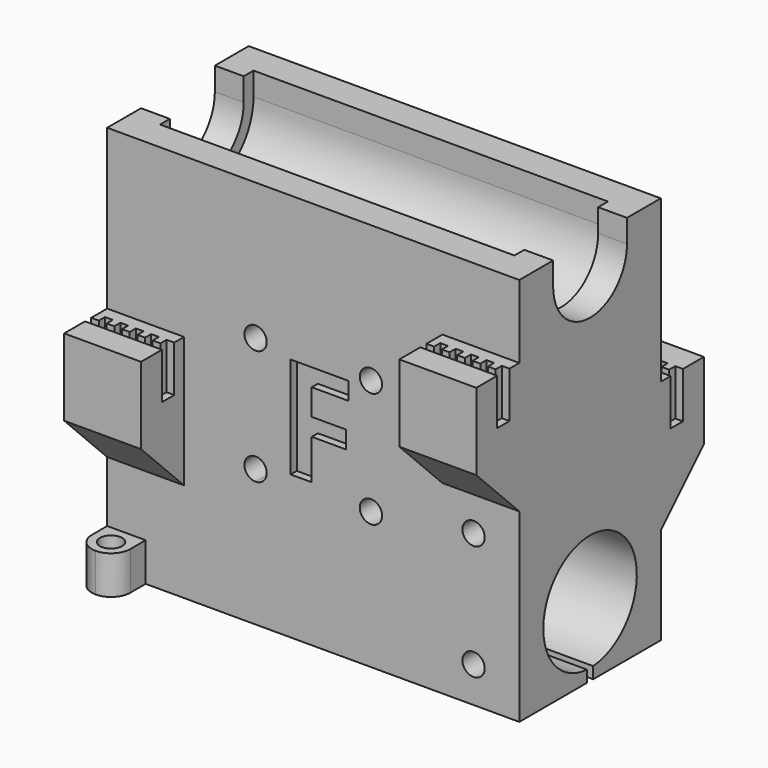
from build123d import *

# Parameters (mm, degrees)
F1_W          = 53.6
F1_H          = 23
F2_DEPTH      = 50.6
F4_DEPTH      = 53.601
F5_DEPTH      = 49.85
F6_DEPTH      = 24.95
F7_DEPTH      = 25.05
F8_DEPTH      = 3.75
F9_W          = 10
F9_H          = 20
F10_DEPTH     = 7
F11_T4_DEPTH  = 61.4336597593
F11_T9_DEPTH  = 61.4336597593
F13_DEPTH     = 6
F15_DEPTH     = 6
F16_W         = 10
F16_H         = 20
F17_DEPTH     = 7
F19_DEPTH     = 6
F21_DEPTH     = 6
F22_T4_DEPTH  = 61.4336597593
F22_T9_DEPTH  = 61.4336597593
F23_R         = 1.45
F24_DEPTH     = 30.001
F25_R         = 1.45
F26_DEPTH     = 5
F27_TEXT_SIZE = 18.4411155982
F28_DEPTH     = 1
F29_W         = 5
F29_H         = 5
F30_DEPTH     = 5
F31_R         = 1.45
F32_DEPTH     = 25
F33_R         = 2.49999


# Not quite as in the source:
# - a fillet or chamfer that OpenCascade refuses, or shapes differently, is made with other operations: its cross-section is extruded or revolved along the edge and cut away or added
# - a fillet or chamfer is up to 0.001 mm smaller than in the source, because OpenCascade refuses the exact size
# - a feature names something its author has since deleted; it is built from what else it names
# - Text() gives the source's letters only with a copy of the font that has no kerning and outlines rounded to 1/6400 em; it was checked with that copy


with BuildPart() as f2:
    # F1 (on Top) → F2 (new body)
    with BuildSketch(Plane.XY):
        with Locations((26.8, 11.5)):
            Rectangle(F1_W, F1_H)
    extrude(amount=F2_DEPTH)

    # F3 (on face) → F4 (cut, through all)
    with BuildSketch(Plane(origin=(0, 0, 0), x_dir=(0, -1, 0), z_dir=(-1, 0, 0))):
        with BuildLine():
            ThreePointArc((-11, 1.5164652041), (-11.5, 1.5), (-12, 1.5164652041))
            Line((-12, 1.5164652041), (-12, 0))
            Line((-12, 0), (-11.5, 0))
            Line((-11.5, 0), (-11, 0))
            Line((-11, 0), (-11, 1.5164652041))
        make_face()
        with BuildLine():
            Line((-11, 1.5164652041), (-12, 1.5164652041))
            ThreePointArc((-12, 1.5164652041), (-11.5, 1.5), (-11, 1.5164652041))
        make_face()
        with BuildLine():
            ThreePointArc((-11, 1.5164652041), (-5.9520273973, 3.9057724347), (-3.9, 9.1))
            ThreePointArc((-3.9, 9.1), (-16.6942275653, 14.6479726027), (-12, 1.5164652041))
            Line((-12, 1.5164652041), (-11, 1.5164652041))
        make_face()
        with BuildLine():
            Line((-5.5, 47.6), (-5.5, 50.6))
            Line((-5.5, 50.6), (-6.3038475773, 50.6))
            ThreePointArc((-6.3038475773, 50.6), (-5.7044450423, 49.1529142706), (-5.5, 47.6))
        make_face()
        with BuildLine():
            Line((-16.6961524227, 50.6), (-17.5, 50.6))
            Line((-17.5, 50.6), (-17.5, 47.6))
            ThreePointArc((-17.5, 47.6), (-17.2955549577, 49.1529142706), (-16.6961524227, 50.6))
        make_face()
        with BuildLine():
            ThreePointArc((-16.6961524227, 50.6), (-17.2955549577, 49.1529142706), (-17.5, 47.6))
            ThreePointArc((-17.5, 47.6), (-11.5, 41.6), (-5.5, 47.6))
            ThreePointArc((-5.5, 47.6), (-5.7044450423, 49.1529142706), (-6.3038475773, 50.6))
            Line((-6.3038475773, 50.6), (-16.6961524227, 50.6))
        make_face()
    extrude(amount=-F4_DEPTH, mode=Mode.SUBTRACT)

    # F3 (on face) → F5 (cut)
    with BuildSketch(Plane(origin=(0, 0, 0), x_dir=(0, -1, 0), z_dir=(-1, 0, 0))):
        with BuildLine():
            ThreePointArc((-18.4828361, 50.6), (-18.9441102343, 49.1314120346), (-19.1, 47.6))
            ThreePointArc((-19.1, 47.6), (-11.5, 40), (-3.9, 47.6))
            ThreePointArc((-3.9, 47.6), (-4.0558897657, 49.1314120346), (-4.5171639, 50.6))
            Line((-4.5171639, 50.6), (-5.5, 50.6))
            Line((-5.5, 50.6), (-5.5, 47.6))
            ThreePointArc((-5.5, 47.6), (-11.5, 41.6), (-17.5, 47.6))
            Line((-17.5, 47.6), (-17.5, 50.6))
            Line((-17.5, 50.6), (-18.4828361, 50.6))
        make_face()
        with BuildLine():
            Line((-18.4828361, 50.6), (-19.1, 50.6))
            Line((-19.1, 50.6), (-19.1, 47.6))
            ThreePointArc((-19.1, 47.6), (-18.9441102343, 49.1314120346), (-18.4828361, 50.6))
        make_face()
        with BuildLine():
            Line((-3.9, 47.6), (-3.9, 50.6))
            Line((-3.9, 50.6), (-4.5171639, 50.6))
            ThreePointArc((-4.5171639, 50.6), (-4.0558897657, 49.1314120346), (-3.9, 47.6))
        make_face()
    extrude(amount=-F5_DEPTH, mode=Mode.SUBTRACT)

    # F3 (on face) → F6 (join)
    with BuildSketch(Plane(origin=(0, 0, 0), x_dir=(0, -1, 0), z_dir=(-1, 0, 0))):
        with BuildLine():
            ThreePointArc((-18.4828361, 50.6), (-18.9441102343, 49.1314120346), (-19.1, 47.6))
            ThreePointArc((-19.1, 47.6), (-11.5, 40), (-3.9, 47.6))
            ThreePointArc((-3.9, 47.6), (-4.0558897657, 49.1314120346), (-4.5171639, 50.6))
            Line((-4.5171639, 50.6), (-5.5, 50.6))
            Line((-5.5, 50.6), (-5.5, 47.6))
            ThreePointArc((-5.5, 47.6), (-11.5, 41.6), (-17.5, 47.6))
            Line((-17.5, 47.6), (-17.5, 50.6))
            Line((-17.5, 50.6), (-18.4828361, 50.6))
        make_face()
        with BuildLine():
            Line((-18.4828361, 50.6), (-19.1, 50.6))
            Line((-19.1, 50.6), (-19.1, 47.6))
            ThreePointArc((-19.1, 47.6), (-18.9441102343, 49.1314120346), (-18.4828361, 50.6))
        make_face()
        with BuildLine():
            Line((-3.9, 47.6), (-3.9, 50.6))
            Line((-3.9, 50.6), (-4.5171639, 50.6))
            ThreePointArc((-4.5171639, 50.6), (-4.0558897657, 49.1314120346), (-3.9, 47.6))
        make_face()
    extrude(amount=-F6_DEPTH)

    # F3 (on face) → F7 (cut)
    with BuildSketch(Plane(origin=(0, 0, 0), x_dir=(0, -1, 0), z_dir=(-1, 0, 0))):
        with BuildLine():
            ThreePointArc((-18.4828361, 50.6), (-18.9441102343, 49.1314120346), (-19.1, 47.6))
            ThreePointArc((-19.1, 47.6), (-11.5, 40), (-3.9, 47.6))
            ThreePointArc((-3.9, 47.6), (-4.0558897657, 49.1314120346), (-4.5171639, 50.6))
            Line((-4.5171639, 50.6), (-5.5, 50.6))
            Line((-5.5, 50.6), (-5.5, 47.6))
            ThreePointArc((-5.5, 47.6), (-11.5, 41.6), (-17.5, 47.6))
            Line((-17.5, 47.6), (-17.5, 50.6))
            Line((-17.5, 50.6), (-18.4828361, 50.6))
        make_face()
        with BuildLine():
            Line((-18.4828361, 50.6), (-19.1, 50.6))
            Line((-19.1, 50.6), (-19.1, 47.6))
            ThreePointArc((-19.1, 47.6), (-18.9441102343, 49.1314120346), (-18.4828361, 50.6))
        make_face()
        with BuildLine():
            Line((-3.9, 47.6), (-3.9, 50.6))
            Line((-3.9, 50.6), (-4.5171639, 50.6))
            ThreePointArc((-4.5171639, 50.6), (-4.0558897657, 49.1314120346), (-3.9, 47.6))
        make_face()
    extrude(amount=-F7_DEPTH, mode=Mode.SUBTRACT)

    # F3 (on face) → F8 (join)
    with BuildSketch(Plane(origin=(0, 0, 0), x_dir=(0, -1, 0), z_dir=(-1, 0, 0))):
        with BuildLine():
            ThreePointArc((-18.4828361, 50.6), (-18.9441102343, 49.1314120346), (-19.1, 47.6))
            ThreePointArc((-19.1, 47.6), (-11.5, 40), (-3.9, 47.6))
            ThreePointArc((-3.9, 47.6), (-4.0558897657, 49.1314120346), (-4.5171639, 50.6))
            Line((-4.5171639, 50.6), (-5.5, 50.6))
            Line((-5.5, 50.6), (-5.5, 47.6))
            ThreePointArc((-5.5, 47.6), (-11.5, 41.6), (-17.5, 47.6))
            Line((-17.5, 47.6), (-17.5, 50.6))
            Line((-17.5, 50.6), (-18.4828361, 50.6))
        make_face()
        with BuildLine():
            Line((-18.4828361, 50.6), (-19.1, 50.6))
            Line((-19.1, 50.6), (-19.1, 47.6))
            ThreePointArc((-19.1, 47.6), (-18.9441102343, 49.1314120346), (-18.4828361, 50.6))
        make_face()
        with BuildLine():
            Line((-3.9, 47.6), (-3.9, 50.6))
            Line((-3.9, 50.6), (-4.5171639, 50.6))
            ThreePointArc((-4.5171639, 50.6), (-4.0558897657, 49.1314120346), (-3.9, 47.6))
        make_face()
    extrude(amount=-F8_DEPTH)

    # F9 (on face) → F10 (join)
    with BuildSketch(Plane.XZ):
        with Locations((5, 19.9)):
            Rectangle(F9_W, F9_H)
        with Locations((48.6, 31.1)):
            Rectangle(F9_W, F9_H)
    extrude(amount=F10_DEPTH)

    # F11: chamfer of 10 on 2 edges, made by hand


with BuildPart() as f11_tool2:
    # F11_s3 → F11_t4 (new body)
    with BuildSketch(Plane.YZ.offset(-25.7168298797)):
        Polygon((3, 9.9), (-7, 19.9), (-7, 9.9), align=None)
    extrude(amount=F11_T4_DEPTH)

    split(bisect_by=Plane.XZ, keep=Keep.TOP)


with BuildPart() as f2_1:
    add(f2.part)

    # F11_t1: cut F11_tool2
    add(f11_tool2.part, mode=Mode.SUBTRACT)


with BuildPart() as f11_tool7:
    # F11_s8 → F11_t9 (new body)
    with BuildSketch(Plane.YZ.offset(17.8831701203)):
        Polygon((3, 21.1), (-7, 31.1), (-7, 21.1), align=None)
    extrude(amount=F11_T9_DEPTH)

    split(bisect_by=Plane.XZ, keep=Keep.TOP)


with BuildPart() as f2_2:
    add(f2_1.part)

    # F11_t6: cut F11_tool7
    add(f11_tool7.part, mode=Mode.SUBTRACT)

    # F12 (on face) → F13 (cut)
    with BuildSketch(Plane.XY.offset(29.9)):
        Polygon((0, -2.6), (0, -3.6), (10, -3.6), (10, -2.6), (10, -1.6), (9, -1.6), (9, -2.6), (8, -2.6), (8, -1.6), (7, -1.6), (7, -2.6), (6, -2.6), (6, -1.6), (5.2958247252, -1.6), (5, -1.6), (5, -2.6), (4, -2.6), (4, -1.6), (3, -1.6), (3, -2.6), (2, -2.6), (2, -1.6), (1, -1.6), (1, -2.6), align=None)
    extrude(amount=-F13_DEPTH, mode=Mode.SUBTRACT)

    # F14 (on face) → F15 (cut)
    with BuildSketch(Plane.XY.offset(41.1)):
        Polygon((43.6, -2.6), (43.6, -3.6), (53.6, -3.6), (53.6, -2.6), (53.6, -1.6), (52.6, -1.6), (52.6, -2.6), (51.6, -2.6), (51.6, -1.6), (50.6, -1.6), (50.6, -2.6), (49.6, -2.6), (49.6, -1.6), (48.8349036932, -1.6), (48.6, -1.6), (48.6, -2.6), (47.6, -2.6), (47.6, -1.6), (46.6, -1.6), (46.6, -2.6), (45.6, -2.6), (45.6, -1.6), (44.6, -1.6), (44.6, -2.6), align=None)
    extrude(amount=-F15_DEPTH, mode=Mode.SUBTRACT)

    # F16 (on face) → F17 (join)
    with BuildSketch(Plane(origin=(0, 23, 0), x_dir=(-1, 0, 0), z_dir=(0, 1, 0))):
        with Locations((-48.6, 19.6)):
            Rectangle(F16_W, F16_H)
        with Locations((-5, 31.1)):
            Rectangle(F16_W, F16_H)
    extrude(amount=F17_DEPTH)

    # F18 (on face) → F19 (cut)
    with BuildSketch(Plane.XY.offset(29.6)):
        Polygon((43.6, 25.6), (43.6, 24.6), (48.6, 24.6), (53.6, 24.6), (53.6, 25.6), (53.6, 26.6), (52.6, 26.6), (52.6, 25.6), (51.6, 25.6), (51.6, 26.6), (50.6, 26.6), (50.6, 25.6), (49.6, 25.6), (49.6, 26.6), (48.6, 26.6), (48.6, 25.6), (47.6, 25.6), (47.6, 26.6), (46.6, 26.6), (46.6, 25.6), (45.6, 25.6), (45.6, 26.6), (44.6, 26.6), (44.6, 25.6), align=None)
    extrude(amount=-F19_DEPTH, mode=Mode.SUBTRACT)

    # F20 (on face) → F21 (cut)
    with BuildSketch(Plane.XY.offset(41.1)):
        Polygon((7, 25.6), (6, 25.6), (6, 26.6), (5, 26.6), (5, 25.6), (4, 25.6), (4, 26.6), (3, 26.6), (3, 25.6), (2, 25.6), (2, 26.6), (1, 26.6), (1, 25.6), (0, 25.6), (0, 24.6), (5, 24.6), (10, 24.6), (10, 25.6), (10, 26.6), (9, 26.6), (9, 25.6), (8, 25.6), (8, 26.6), (7, 26.6), align=None)
    extrude(amount=-F21_DEPTH, mode=Mode.SUBTRACT)

    # F22: chamfer of 10 on 2 edges, made by hand


with BuildPart() as f22_tool2:
    # F22_s3 → F22_t4 (new body)
    with BuildSketch(Plane.YZ.offset(35.7168298797)):
        Polygon((30, 31.1), (20, 21.1), (30, 21.1), align=None)
    extrude(amount=-F22_T4_DEPTH)

    split(bisect_by=Plane.XZ.offset(-23), keep=Keep.BOTTOM)


with BuildPart() as f2_3:
    add(f2_2.part)

    # F22_t1: cut F22_tool2
    add(f22_tool2.part, mode=Mode.SUBTRACT)


with BuildPart() as f22_tool7:
    # F22_s8 → F22_t9 (new body)
    with BuildSketch(Plane.YZ.offset(79.3168298797)):
        Polygon((20, 9.6), (30, 19.6), (30, 9.6), align=None)
    extrude(amount=-F22_T9_DEPTH)

    split(bisect_by=Plane.XZ.offset(-23), keep=Keep.BOTTOM)


with BuildPart() as f2_4:
    add(f2_3.part)

    # F22_t6: cut F22_tool7
    add(f22_tool7.part, mode=Mode.SUBTRACT)

    # F23 (on face) → F24 (cut, through all)
    with BuildSketch(Plane.XZ):
        with BuildLine():
            ThreePointArc((17.85, 32.8), (19.3, 31.35), (20.75, 32.8))
            ThreePointArc((20.75, 32.8), (19.3, 34.25), (17.85, 32.8))
        make_face()
        with BuildLine():
            ThreePointArc((35.75, 32.8), (35.3253048327, 33.8253048327), (34.3, 34.25))
            ThreePointArc((34.3, 34.25), (33.2746951673, 31.7746951673), (35.75, 32.8))
        make_face()
        with BuildLine():
            ThreePointArc((20.75, 17.8), (18.2746951673, 18.8253048327), (19.3, 16.35))
            ThreePointArc((19.3, 16.35), (20.3253048327, 16.7746951673), (20.75, 17.8))
        make_face()
        with Locations((34.3, 17.8)):
            Circle(F23_R)
    extrude(amount=-F24_DEPTH, mode=Mode.SUBTRACT)

    # F25 (on face) → F26 (cut)
    with BuildSketch(Plane.XZ):
        with Locations((47.65, 19.65)):
            Circle(F25_R)
        with Locations((47.65, 4.65)):
            Circle(F25_R)
    extrude(amount=-F26_DEPTH, mode=Mode.SUBTRACT)

    # F27 (on face) → F28 (cut)
    with BuildSketch(Plane.XZ):
        with Locations((22.1983653734, 18.6611983846)):
            Text('F', F27_TEXT_SIZE, font='Open Sans', font_style=FontStyle.BOLD, text_align=(TextAlign.LEFT, TextAlign.BOTTOM))
    extrude(amount=-F28_DEPTH, mode=Mode.SUBTRACT)

    # F29 (on face) → F30 (join)
    with BuildSketch(Plane.XZ):
        with Locations((2.5, 2.5)):
            Rectangle(F29_W, F29_H)
    extrude(amount=F30_DEPTH)

    # F31 (on face) → F32 (cut)
    with BuildSketch(Plane.XY.offset(5)):
        with Locations((2.5, -2.5)):
            Circle(F31_R)
    extrude(amount=-F32_DEPTH, mode=Mode.SUBTRACT)

    # F33 (radius 2.5 in the source; OpenCascade refuses exactly that, so slightly less here)
    f33_edges = [f2_4.edges().sort_by_distance(p)[0] for p in [
        (0, -5, 2.5),
        (5, -5, 2.5),
    ]]
    fillet(f33_edges, radius=F33_R)


solid = f2_4.part
